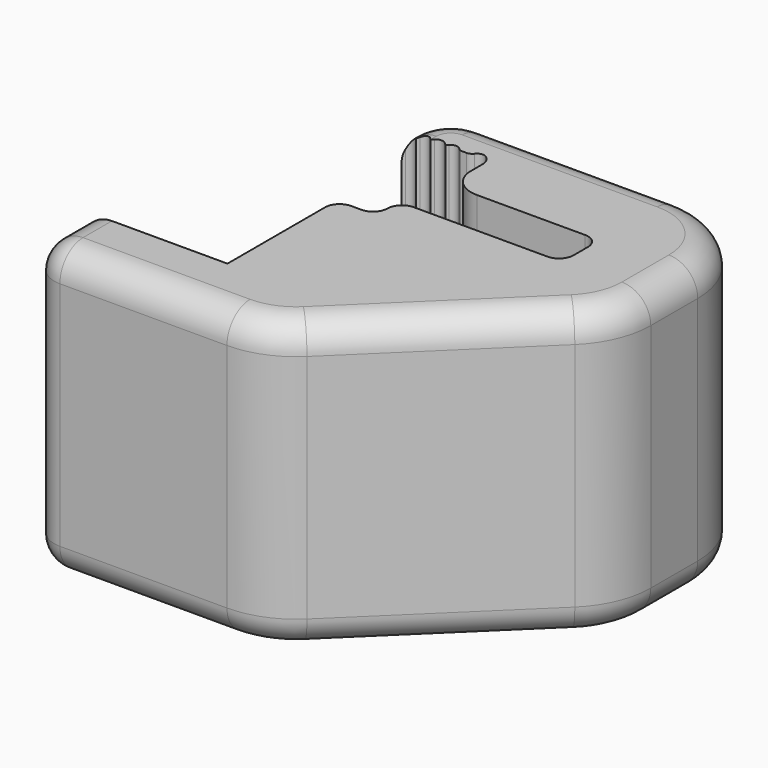
from build123d import *

# Parameters (mm, degrees)
F1_DEPTH = 20
F2_R     = 2


# Not quite as in the source:
# - a feature names something its author has since deleted; it is built from what else it names


with BuildPart() as f1:
    # F0 (on Top) → F1 (new body)
    with BuildSketch(Plane.XY):
        with BuildLine():
            ThreePointArc((-33.4013422072, 19.5177844279), (-33.1069150162, 19.1649980234), (-33.0013422072, 18.7177844279))
            Line((-33.0013422072, 18.7177844279), (-33.0013422072, 17.7177844279))
            ThreePointArc((-33.0013422072, 17.7177844279), (-32.4155557696, 16.3035708655), (-31.0013422072, 15.7177844279))
            Line((-31.0013422072, 15.7177844279), (-23.5013422072, 15.7177844279))
            ThreePointArc((-23.5013422072, 15.7177844279), (-22.794235426, 15.424891209), (-22.5013422072, 14.7177844279))
            Line((-22.5013422072, 14.7177844279), (-22.5013422072, 13.4677844279))
            ThreePointArc((-22.5013422072, 13.4677844279), (-22.794235426, 12.7606776467), (-23.5013422072, 12.4677844279))
            Line((-23.5013422072, 12.4677844279), (-32.781970528, 12.4677844279))
            ThreePointArc((-32.781970528, 12.4677844279), (-33.4890773091, 12.174891209), (-33.781970528, 11.4677844279))
            ThreePointArc((-33.781970528, 11.4677844279), (-34.0748637468, 10.7606776467), (-34.781970528, 10.4677844279))
            Line((-34.781970528, 10.4677844279), (-35.5013422072, 10.4677844279))
            ThreePointArc((-35.5013422072, 10.4677844279), (-36.2084489884, 10.174891209), (-36.5013422072, 9.4677844279))
            Line((-36.5013422072, 9.4677844279), (-36.5013422072, 2.9677844279))
            Line((-36.5013422072, 2.9677844279), (-36.5013422072, 1.0177844279))
            Line((-36.5013422072, 1.0177844279), (-38.5013422072, 1.0177844279))
            Line((-38.5013422072, 1.0177844279), (-46.5013422072, 1.0177844279))
            Line((-46.5013422072, 1.0177844279), (-46.5013422072, 0.5177844279))
            Line((-46.5013422072, 0.5177844279), (-46.5013422072, -1.4822155721))
            ThreePointArc((-46.5013422072, -1.4822155721), (-45.9155557696, -2.8964291345), (-44.5013422072, -3.4822155721))
            Line((-44.5013422072, -3.4822155721), (-32.935840724, -3.4822155721))
            ThreePointArc((-32.935840724, -3.4822155721), (-30.679965917, -3.0419843493), (-28.7551266184, -1.7858918573))
            Line((-28.7551266184, -1.7858918573), (-18.3206281016, 8.3504781304))
            ThreePointArc((-18.3206281016, 8.3504781304), (-16.9748476295, 10.3179485849), (-16.5013422072, 12.6541544156))
            Line((-16.5013422072, 12.6541544156), (-16.5013422072, 16.7177844279))
            ThreePointArc((-16.5013422072, 16.7177844279), (-18.2587015201, 20.960425115), (-22.5013422072, 22.7177844279))
            Line((-22.5013422072, 22.7177844279), (-36.0013422072, 22.7177844279))
            ThreePointArc((-36.0013422072, 22.7177844279), (-38.1226625508, 21.8391047714), (-39.0013422072, 19.7177844279))
            Line((-39.0013422072, 19.7177844279), (-39.0013422072, 19.2177844279))
            Line((-39.0013422072, 19.2177844279), (-38.8548955978, 19.3642310373))
            ThreePointArc((-38.8548955978, 19.3642310373), (-38.5013422072, 19.5106776467), (-38.1477888166, 19.3642310373))
            Line((-38.1477888166, 19.3642310373), (-38.0013422072, 19.2177844279))
            Line((-38.0013422072, 19.2177844279), (-37.8548955978, 19.3642310373))
            ThreePointArc((-37.8548955978, 19.3642310373), (-37.5013422072, 19.5106776467), (-37.1477888166, 19.3642310373))
            Line((-37.1477888166, 19.3642310373), (-37.0013422072, 19.2177844279))
            Line((-37.0013422072, 19.2177844279), (-36.8463774903, 19.3727491447))
            ThreePointArc((-36.8463774903, 19.3727491447), (-36.498920301, 19.5191585891), (-36.1479965135, 19.3812647196))
            Line((-36.1479965135, 19.3812647196), (-35.9763422072, 19.2177844279))
            Line((-35.9763422072, 19.2177844279), (-35.8449793172, 19.3557154623))
            ThreePointArc((-35.8449793172, 19.3557154623), (-35.4951018479, 19.5107392214), (-35.1380827655, 19.3729568416))
            Line((-35.1380827655, 19.3729568416), (-35.0041172482, 19.2453706347))
            ThreePointArc((-35.0041172482, 19.2453706347), (-34.9722907986, 19.2249367588), (-34.935151731, 19.2177844279))
            Line((-34.935151731, 19.2177844279), (-34.5013422072, 19.2177844279))
            ThreePointArc((-34.5013422072, 19.2177844279), (-34.2777354094, 19.2705708324), (-34.1013422072, 19.4177844279))
            ThreePointArc((-34.1013422072, 19.4177844279), (-33.7720528853, 19.6127591747), (-33.4013422072, 19.5177844279))
        make_face()
    extrude(amount=F1_DEPTH)

    # F2
    f2_edges = [f1.edges().sort_by_distance(p)[0] for p in [
        (-29.251342, 22.717784, 20),
        (-29.251342, 22.717784, 0),
    ]]
    fillet(f2_edges, radius=F2_R)


solid = f1.part
